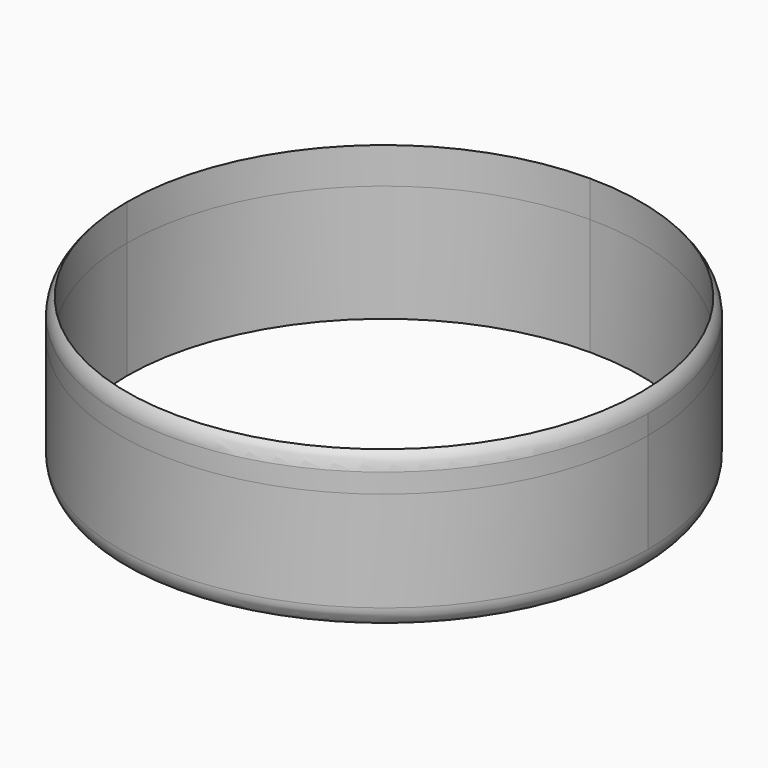
from build123d import *

# Parameters (mm, degrees)
F1_DEPTH = 7.62
F2_DEPTH = 24.638


# Not quite as in the source:
# - a fillet or chamfer that OpenCascade refuses, or shapes differently, is made with other operations: its cross-section is extruded or revolved along the edge and cut away or added


with BuildPart() as f1:
    # F0 (on Top) → F1 (new body)
    with BuildSketch(Plane.XY):
        with BuildLine():
            ThreePointArc((55.6514, 0), (39.3514823225, 39.3514823225), (0, 55.6514))
            ThreePointArc((0, 55.6514), (-39.3514823225, -39.3514823225), (55.6514, 0))
        make_face()
        with BuildLine():
            ThreePointArc((0, 54.229), (38.345693637, 38.345693637), (54.229, 0))
            ThreePointArc((54.229, 0), (38.345693637, -38.345693637), (0, -54.229))
            ThreePointArc((0, -54.229), (-38.345693637, -38.345693637), (-54.229, 0))
            ThreePointArc((-54.229, 0), (-38.345693637, 38.345693637), (0, 54.229))
        make_face(mode=Mode.SUBTRACT)
    extrude(amount=F1_DEPTH)

    # F0 (on Top) → F2 (join)
    with BuildSketch(Plane.XY):
        with BuildLine():
            ThreePointArc((55.6514, 0), (39.3514823225, 39.3514823225), (0, 55.6514))
            ThreePointArc((0, 55.6514), (-39.3514823225, -39.3514823225), (55.6514, 0))
        make_face()
        with BuildLine():
            ThreePointArc((0, 54.229), (38.345693637, 38.345693637), (54.229, 0))
            ThreePointArc((54.229, 0), (38.345693637, -38.345693637), (0, -54.229))
            ThreePointArc((0, -54.229), (-38.345693637, -38.345693637), (-54.229, 0))
            ThreePointArc((-54.229, 0), (-38.345693637, 38.345693637), (0, 54.229))
        make_face(mode=Mode.SUBTRACT)
    extrude(amount=-F2_DEPTH)

    # F3: fillet of radius 5.08 on 2 edges, made by hand

    # F3_s1 → F3_t2 (revolve, cut)
    with BuildSketch(Plane.XZ):
        with BuildLine():
            ThreePointArc((55.6514, 4.0946117604), (55.2823981957, 5.9953737129), (54.229, 7.62))
            Line((54.229, 7.62), (55.6514, 7.62))
            Line((55.6514, 7.62), (55.6514, 4.0946117604))
        make_face()
    revolve(axis=Axis((0, 0, 7.62), (0, 0, -1)), mode=Mode.SUBTRACT)

    # F3_s3 → F3_t4 (revolve, cut)
    with BuildSketch(Plane.XZ):
        with BuildLine():
            ThreePointArc((55.6514, -21.1126117604), (55.2823981957, -23.0133737129), (54.229, -24.638))
            Line((54.229, -24.638), (55.6514, -24.638))
            Line((55.6514, -24.638), (55.6514, -21.1126117604))
        make_face()
    revolve(axis=Axis((0, 0, -24.638), (0, 0, 1)), mode=Mode.SUBTRACT)


solid = f1.part
